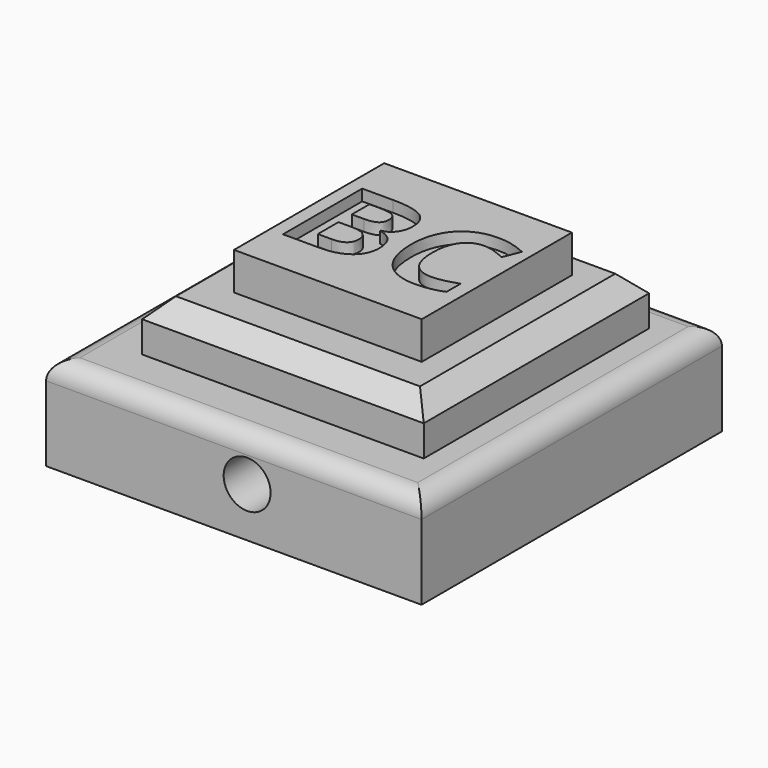
from build123d import *

# Parameters (mm, degrees)
F0_W          = 101.6
F0_H          = 101.6
F1_DEPTH      = 25.4
F2_W          = 76.2
F2_H          = 76.2
F3_DEPTH      = 38.862
F4_W          = 50.8
F4_H          = 50.8
F5_DEPTH      = 49.022
F6_R          = 6.35
F7_DEPTH      = 154.432
F8_SIZE       = 5.08
F9_R          = 5.08
F10_TEXT_SIZE = 37.52905565
F11_DEPTH     = 3.048


# Not quite as in the source:
# - Text() gives the source's letters only with a copy of the font that has no kerning and outlines rounded to 1/6400 em; it was checked with that copy


with BuildPart() as f1:
    # F0 (on Top) → F1 (new body)
    with BuildSketch(Plane.XY):
        with Locations((50.8, 50.8)):
            Rectangle(F0_W, F0_H)
    extrude(amount=F1_DEPTH)

    # F2 (on Top) → F3 (join)
    with BuildSketch(Plane.XY):
        with Locations((52.5188283063, 52.5730509126)):
            Rectangle(F2_W, F2_H)
    extrude(amount=F3_DEPTH)

    # F4 (on Top) → F5 (join)
    with BuildSketch(Plane.XY):
        with Locations((53.4203359857, 53.9367885005)):
            Rectangle(F4_W, F4_H)
    extrude(amount=F5_DEPTH)

    # F6 (on Front) → F7 (cut)
    with BuildSketch(Plane.XZ):
        with Locations((54.405618459, 13.3619941771)):
            Circle(F6_R)
    extrude(amount=-F7_DEPTH, mode=Mode.SUBTRACT)

    # F8
    f8_edges = [f1.edges().sort_by_distance(p)[0] for p in [
        (90.618828, 52.573051, 38.862),
        (52.518828, 14.473051, 38.862),
        (14.418828, 52.573051, 38.862),
        (52.518828, 90.673051, 38.862),
    ]]
    chamfer(f8_edges, length=F8_SIZE)

    # F9
    f9_edges = [f1.edges().sort_by_distance(p)[0] for p in [
        (50.8, 0, 25.4),
        (0, 50.8, 25.4),
        (101.6, 50.8, 25.4),
        (50.8, 101.6, 25.4),
    ]]
    fillet(f9_edges, radius=F9_R)

    # F10 (on face) → F11 (cut)
    with BuildSketch(Plane.XY.offset(49.022)):
        with Locations((28.2744262367, 40.571231395)):
            Text('BC', F10_TEXT_SIZE, font='Open Sans', font_style=FontStyle.BOLD, text_align=(TextAlign.LEFT, TextAlign.BOTTOM))
    extrude(amount=-F11_DEPTH, mode=Mode.SUBTRACT)


solid = f1.part
